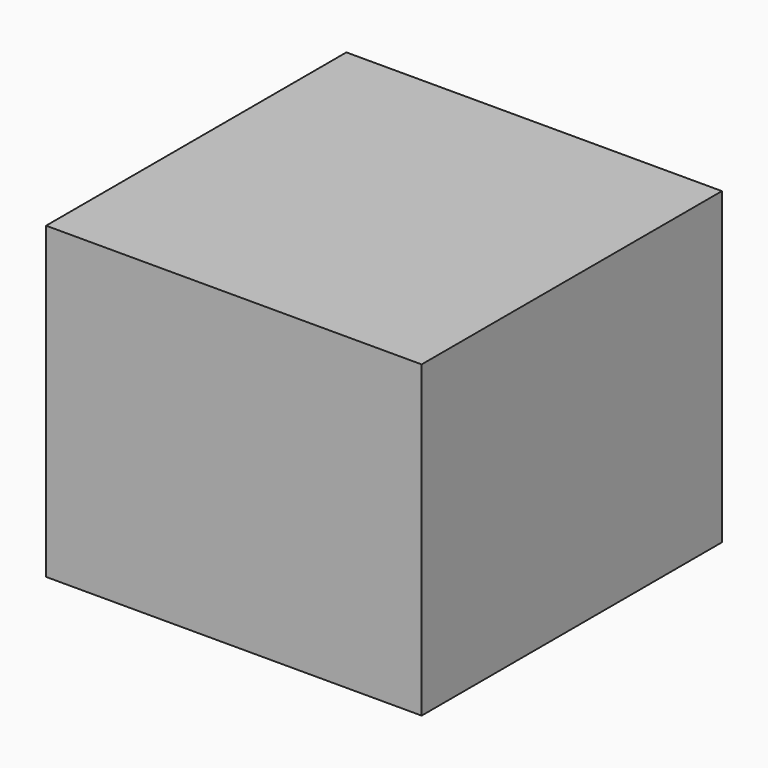
from build123d import *

# Parameters (mm, degrees)
F0_W     = 111.8212044239
F0_H     = 92.0662023127
F1_DEPTH = 111.76
F3_DEPTH = 240


# Not quite as in the source:
# - an extrude ends at something that could not be found from the text; its depth is read off the source's solid


with BuildPart() as f1:
    # F0 (on Front) → F1 (new body)
    with BuildSketch(Plane.XZ):
        with Locations((1.8074549735, 6.1422567815)):
            Rectangle(F0_W, F0_H)
    extrude(amount=F1_DEPTH)

    # F2 (on face) → F3 (cut, through all)
    with BuildSketch(Plane(origin=(0, 0, 0), x_dir=(-1, 0, 0), z_dir=(0, 1, 0))):
        with BuildLine():
            ThreePointArc((-3.9819494155, 18.9731204628), (-12.2196415277, -15.0504346175), (19.3864700562, 0))
            ThreePointArc((19.3864700562, 0), (17.5745341676, 8.1835792924), (12.4774278386, 14.8374194446))
            ThreePointArc((12.4774278386, 14.8374194446), (13.0904581477, 12.8344345243), (13.297498461, 10.7499947771))
            ThreePointArc((13.297498461, 10.7499947771), (-1.8522784042, 1.1818299197), (-3.9819494155, 18.9731204628))
        make_face()
    extrude(amount=F3_DEPTH, mode=Mode.SUBTRACT)


solid = f1.part
